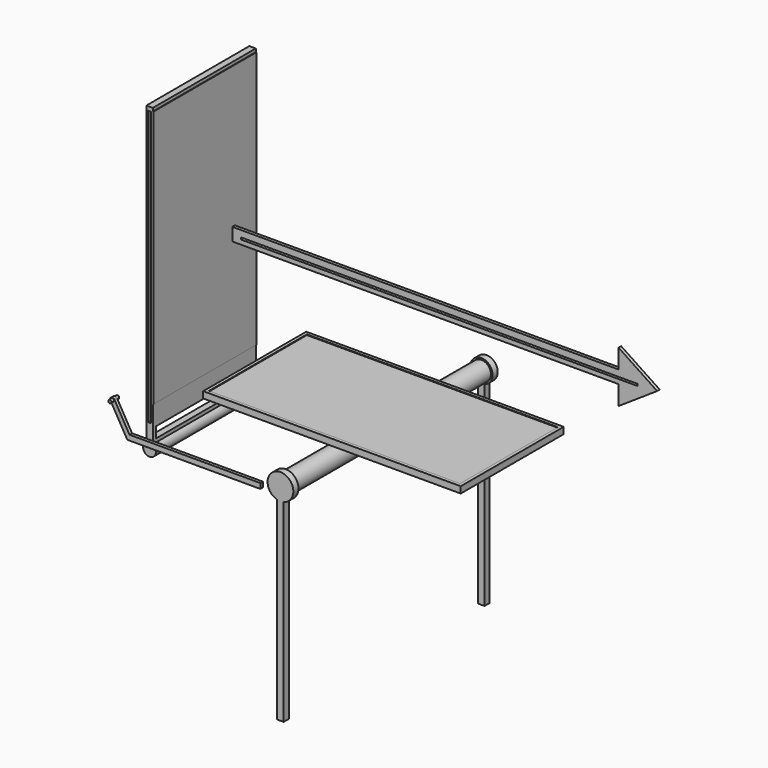
from build123d import *

# Parameters (mm, degrees)
F0_W           = 2000
F0_H           = 1000
F1_DEPTH       = 25
F2_W           = 1950
F2_H           = 950
F4_DEPTH       = 5
F5_R           = 75
F6_DEPTH       = 1000
F7_R           = 100
F7_R_2         = 75
F8_DEPTH       = 50
F9_W           = 50
F9_H           = 1600
F10_DEPTH      = 50
F11_R          = 87.5
F11_R_2        = 75
F12_DEPTH      = 50
F13_W          = 50
F13_H          = 1600
F14_DEPTH      = 50
F16_DEPTH      = 500
F17_W          = 25.1
F17_H          = 2129.8030083389
F18_DEPTH      = 25
F20_W          = 936.323851347
F20_H          = 83.1241309643
F21_DEPTH      = 75.001
F22_W          = 1000
F22_H          = 2000
F23_DEPTH      = 4
F24_R          = 12.5
F25_DEPTH      = 25
F26_R          = 12.5
F27_DEPTH      = 50
F27_DEPTH_BACK = 25
F29_DEPTH      = 12.5
F31_W          = 3080.738902092
F31_H          = 15.1523351669
F32_DEPTH      = 1012.501
F33_R          = 25
F34_DEPTH      = 50
F35_W          = 50
F35_H          = 50
F36_DEPTH      = 50


# Not quite as in the source:
# - a feature names something its author has since deleted; it is built from what else it names


with BuildPart() as f1:
    # F0 (on Top) → F1 (new body, symmetric)
    with BuildSketch(Plane.XY):
        Rectangle(F0_W, F0_H)
    extrude(amount=F1_DEPTH, both=True)

    # F2 (on face) → F4 (cut)
    with BuildSketch(Plane.XY.offset(25)):
        Rectangle(F2_W, F2_H)
    extrude(amount=-F4_DEPTH, mode=Mode.SUBTRACT)

    # F5 (on Front) → F6 (join, symmetric)
    with BuildSketch(Plane.XZ):
        with Locations((0, -100)):
            Circle(F5_R)
    extrude(amount=F6_DEPTH, both=True)

    # F7 (on face) → F8 (join)
    with BuildSketch(Plane.XZ.offset(1000)):
        with Locations((0, -100)):
            Circle(F7_R)
        with Locations((0, -100)):
            Circle(F7_R_2, mode=Mode.SUBTRACT)
    extrude(amount=-F8_DEPTH)

    # F9 (on face) → F10 (join)
    with BuildSketch(Plane.XZ.offset(1000)):
        with Locations((0, -900)):
            Rectangle(F9_W, F9_H)
    extrude(amount=-F10_DEPTH)

    # F11 (on face) → F12 (join)
    with BuildSketch(Plane(origin=(0, 1000, 0), x_dir=(-1, 0, 0), z_dir=(0, 1, 0))):
        with Locations((0, -100)):
            Circle(F11_R)
        with Locations((0, -100)):
            Circle(F11_R_2, mode=Mode.SUBTRACT)
    extrude(amount=-F12_DEPTH)

    # F13 (on face) → F14 (join)
    with BuildSketch(Plane(origin=(0, 1000, 0), x_dir=(-1, 0, 0), z_dir=(0, 1, 0))):
        with Locations((0, -900)):
            Rectangle(F13_W, F13_H)
    extrude(amount=-F14_DEPTH)


with BuildPart() as f16:
    # F15 (on Front) → F16 (new body, symmetric)
    with BuildSketch(Plane.XZ):
        with BuildLine():
            Line((-1441.7065932193, 1834.076336483), (-1441.7065932193, -465.923663517))
            ThreePointArc((-1441.7065932193, -465.923663517), (-1416.7065932193, -559.2249337063), (-1391.7065932193, -465.923663517))
            Line((-1391.7065932193, -465.923663517), (-1391.7065932193, 1834.076336483))
            Line((-1391.7065932193, 1834.076336483), (-1441.7065932193, 1834.076336483))
        make_face()
    extrude(amount=F16_DEPTH, both=True)

    # F17 (on face) → F18 (cut)
    with BuildSketch(Plane.XZ.offset(500)):
        with Locations((-1416.7565932193, 738.5590938225)):
            Rectangle(F17_W, F17_H)
    f18 = extrude(amount=-F18_DEPTH, mode=Mode.SUBTRACT)

    # F19: F18 across plane
    add(f18.mirror(Plane.XZ), mode=Mode.SUBTRACT)

    # F20 (on face) → F21 (cut, through all)
    with BuildSketch(Plane.YZ.offset(-1391.7065932193)):
        with Locations((-2.4584084749, -396.9483524561)):
            Rectangle(F20_W, F20_H)
    extrude(amount=-F21_DEPTH, mode=Mode.SUBTRACT)

    # F22 (on face) → F23 (join)
    with BuildSketch(Plane.YZ.offset(-1391.7065932193)):
        with Locations((0, 809.076336483)):
            Rectangle(F22_W, F22_H)
    extrude(amount=F23_DEPTH)


with BuildPart() as f25:
    # F24 (on face) → F25 (new body)
    with BuildSketch(Plane.XZ.offset(1000)):
        with BuildLine():
            Line((-136.3898057708, -149.4357743859), (-136.3898057708, -109.4357743859))
            Line((-136.3898057708, -109.4357743859), (-1152.4184524861, -109.4357743859))
            Line((-1152.4184524861, -109.4357743859), (-1270.6376314163, 95.3258499503))
            ThreePointArc((-1270.6376314163, 95.3258499503), (-1294.3903554093, 99.7139583837), (-1300.0246226155, 76.2256117888))
            Line((-1300.0246226155, 76.2256117888), (-1169.7389605618, -149.4357743859))
            Line((-1169.7389605618, -149.4357743859), (-136.3898057708, -149.4357743859))
        make_face()
        with Locations((-1284.8269364284, 85)):
            Circle(F24_R, mode=Mode.SUBTRACT)
    extrude(amount=F25_DEPTH)

    # F26 (on face) → F27 (join, two sides)
    with BuildSketch(Plane.XZ.offset(1025)) as f27_sk:
        with Locations((-1284.8269364284, 85)):
            Circle(F26_R)
    extrude(amount=-F27_DEPTH)
    extrude(f27_sk.sketch, amount=F27_DEPTH_BACK)


with BuildPart() as f29:
    # F28 (on Front) → F29 (new body, symmetric)
    with BuildSketch(Plane.XZ):
        Polygon((-1164.3936634064, 897.0192074776), (-1164.3936634064, 797.0192074776), (1835.6063365936, 797.0192074776), (1835.6063365936, 647.0192074776), (2135.6063365936, 847.0192074776), (1835.6063365936, 1047.0192074776), (1835.6063365936, 897.0192074776), align=None)
    extrude(amount=F29_DEPTH, both=True)

    # F31 (on face) → F32 (cut, through all)
    with BuildSketch(Plane.XZ.offset(12.5)):
        with Locations((442.9072737694, 839.4430398941)):
            Rectangle(F31_W, F31_H)
    extrude(amount=-F32_DEPTH, mode=Mode.SUBTRACT)


with BuildPart() as f34:
    # F33 (on Front) → F34 (new body, symmetric)
    with BuildSketch(Plane.XZ):
        with Locations((-900.4946947098, 269.2202627659)):
            Circle(F33_R)
    extrude(amount=F34_DEPTH, both=True)


with BuildPart() as f36:
    # F35 (on Front) → F36 (new body, symmetric)
    with BuildSketch(Plane.XZ):
        with Locations((-907.7636889409, -156.4750745893)):
            Rectangle(F35_W, F35_H)
    extrude(amount=F36_DEPTH, both=True)


solid = Compound([f1.part, f16.part, f25.part, f29.part, f36.part])
